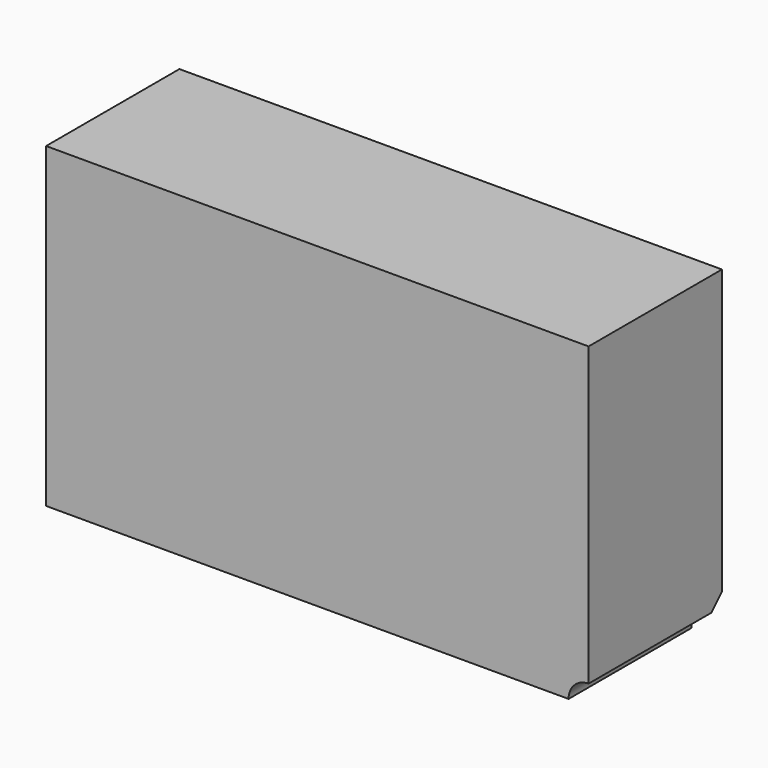
from build123d import *

# Parameters (mm, degrees)
F1_W           = 82.6707333326
F1_H           = 48.286376521
F2_DEPTH       = 25.4
F3_D           = 6.096
F3_CSINK_D     = 10.16
F3_CSINK_ANGLE = 90


# Not quite as in the source:
# - a variable given as a bare number and used for a length is read in inches; the dataset says mm whatever the document's units were


with BuildPart() as f2:
    # F1 (on Front) → F2 (new body)
    with BuildSketch(Plane.XZ):
        with Locations((-41.3353666663, 8.0742510036)):
            Rectangle(F1_W, F1_H)
    extrude(amount=F2_DEPTH)

    # F3 (through all)
    with Locations(Plane(origin=(0, 0, 0), x_dir=(1, 0, 0), z_dir=(0, 1, 0))):
        with Locations((0, 16.0689372569)):
            CounterSinkHole(F3_D / 2, F3_CSINK_D / 2, counter_sink_angle=F3_CSINK_ANGLE)


solid = f2.part
